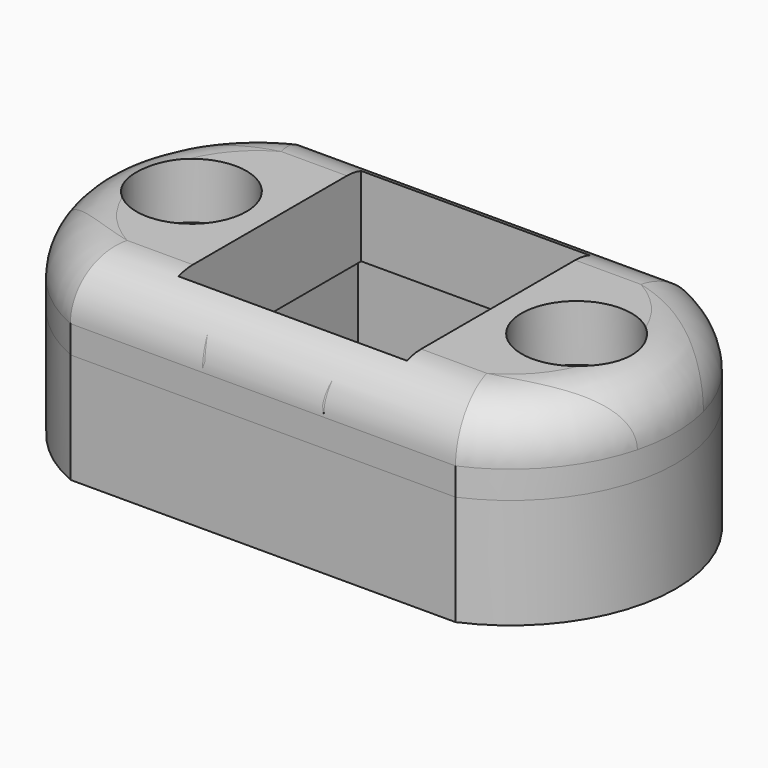
from build123d import *

# Parameters (mm, degrees)
F0_W           = 14
F0_H           = 11
F1_DEPTH       = 4
F2_R           = 1
F2_W           = 9.5
F2_H           = 9.5
F3_DEPTH       = 5
F4_W           = 14
F4_H           = 11
F5_DEPTH       = 3
F6_W           = 8.3
F6_H           = 8.3
F7_DEPTH       = 3
F8_T1_DEPTH    = 24
F8_T6_ANGLE    = 228.4636950683
F8_S7_R        = 2
F8_T8_DEPTH    = 9
F8_S9_R        = 2
F8_T10_DEPTH   = 9
F8_T14_ANGLE   = 228.4636950683
F8_T19_ANGLE   = 228.4636950683
F8_S20_R       = 2
F8_T21_DEPTH   = 9
F8_S22_R       = 2
F8_T23_DEPTH   = 9
F8_T27_ANGLE   = 228.4636950683
F9_D           = 2
F9_DEPTH       = 20
F9_START       = 0.039984
F9_CBORE_D     = 4
F9_CBORE_DEPTH = 2
F9_TIP         = 0.600860619


# Not quite as in the source:
# - a fillet or chamfer that OpenCascade refuses, or shapes differently, is made with other operations: its cross-section is extruded or revolved along the edge and cut away or added


with BuildPart() as f1:
    # F0 (on Top) → F1 (new body)
    with BuildSketch(Plane.XY):
        Rectangle(F0_W, F0_H)
        with BuildLine():
            ThreePointArc((7, -5.5), (10.6020842383, 0), (7, 5.5))
            Line((7, 5.5), (7, -5.5))
        make_face()
        with BuildLine():
            Line((-7, -5.5), (-7, 5.5))
            ThreePointArc((-7, 5.5), (-10.6020842383, 0), (-7, -5.5))
        make_face()
    extrude(amount=F1_DEPTH)

    # F2 (on face) → F3 (cut)
    with BuildSketch(Plane.XY.offset(4)):
        with Locations((-7, 0)):
            Circle(F2_R)
        with Locations((7, 0)):
            Circle(F2_R)
        Rectangle(F2_W, F2_H)
    extrude(amount=-F3_DEPTH, mode=Mode.SUBTRACT)


with BuildPart() as f5:
    # F4 (on face) → F5 (new body)
    with BuildSketch(Plane.XY.offset(4)):
        Rectangle(F4_W, F4_H)
        with BuildLine():
            ThreePointArc((7, -5.5), (10.6020842383, 0), (7, 5.5))
            Line((7, 5.5), (7, -5.5))
        make_face()
        with BuildLine():
            Line((-7, -5.5), (-7, 5.5))
            ThreePointArc((-7, 5.5), (-10.6020842383, 0), (-7, -5.5))
        make_face()
    extrude(amount=F5_DEPTH)

    # F6 (on face) → F7 (cut)
    with BuildSketch(Plane.XY.offset(7)):
        Rectangle(F6_W, F6_H)
    extrude(amount=-F7_DEPTH, mode=Mode.SUBTRACT)

    # F8: fillet of radius 2 on 4 edges, made by hand

    # F8_s2 → F8_t1 (cut)
    with BuildSketch(Plane.YZ.offset(-12)):
        with BuildLine():
            ThreePointArc((5.5, 5), (4.9142135624, 6.4142135624), (3.5, 7))
            Line((3.5, 7), (5.5, 7))
            Line((5.5, 7), (5.5, 5))
        make_face()
        with BuildLine():
            ThreePointArc((-3.5, 7), (-4.9142135624, 6.4142135624), (-5.5, 5))
            Line((-5.5, 5), (-5.5, 7))
            Line((-5.5, 7), (-3.5, 7))
        make_face()
    extrude(amount=F8_T1_DEPTH, mode=Mode.SUBTRACT)


with BuildPart() as f8_tool4:
    # F8_s5 → F8_t6 (revolve)
    with BuildSketch(Plane(origin=(3.8268504556, -1.7224121907, 0), x_dir=(0, 0, 1), z_dir=(-0.9118921219, 0.4104299673, 0))):
        with BuildLine():
            ThreePointArc((5, -4.1111667166), (6.4142135624, -3.525380279), (7, -2.1111667166))
            Line((7, -2.1111667166), (7, -4.1111667166))
            Line((7, -4.1111667166), (5, -4.1111667166))
        make_face()
    revolve(axis=Axis((4.6020842383, 0, 7), (0, 0, 1)), revolution_arc=F8_T6_ANGLE)

    # F8_s7 → F8_t8 (cut, symmetric)
    with BuildSketch(Plane.YZ.offset(6.3)):
        with Locations((3.5, 5)):
            Circle(F8_S7_R)
    extrude(amount=F8_T8_DEPTH, both=True, mode=Mode.SUBTRACT)

    # F8_s9 → F8_t10 (cut, symmetric)
    with BuildSketch(Plane.YZ.offset(6.3)):
        with Locations((-3.5, 5)):
            Circle(F8_S9_R)
    extrude(amount=F8_T10_DEPTH, both=True, mode=Mode.SUBTRACT)


with BuildPart() as f5_1:
    add(f5.part)

    # F8_t3: cut F8_tool4
    add(f8_tool4.part, mode=Mode.SUBTRACT)


with BuildPart() as f8_tool12:
    # F8_s13 → F8_t14 (revolve)
    with BuildSketch(Plane(origin=(3.8268504556, -1.7224121907, 0), x_dir=(0, 0, 1), z_dir=(-0.9118921219, 0.4104299673, 0))):
        with BuildLine():
            ThreePointArc((5, -4.1111667166), (6.4142135624, -3.525380279), (7, -2.1111667166))
            Line((7, -2.1111667166), (7, -4.1111667166))
            Line((7, -4.1111667166), (5, -4.1111667166))
        make_face()
    revolve(axis=Axis((4.6020842383, 0, 7), (0, 0, 1)), revolution_arc=F8_T14_ANGLE)

    split(bisect_by=Plane.YZ.offset(4.15), keep=Keep.TOP)


with BuildPart() as f5_2:
    add(f5_1.part)

    # F8_t11: cut F8_tool12
    add(f8_tool12.part, mode=Mode.SUBTRACT)


with BuildPart() as f8_tool17:
    # F8_s18 → F8_t19 (revolve)
    with BuildSketch(Plane(origin=(-3.8268504556, 1.7224121907, 0), x_dir=(0, 0, 1), z_dir=(0.9118921219, -0.4104299673, 0))):
        with BuildLine():
            ThreePointArc((5, -4.1111667166), (6.4142135624, -3.525380279), (7, -2.1111667166))
            Line((7, -2.1111667166), (7, -4.1111667166))
            Line((7, -4.1111667166), (5, -4.1111667166))
        make_face()
    revolve(axis=Axis((-4.6020842383, 0, 7), (0, 0, 1)), revolution_arc=F8_T19_ANGLE)

    # F8_s20 → F8_t21 (cut, symmetric)
    with BuildSketch(Plane.YZ.offset(-6.3)):
        with Locations((3.5, 5)):
            Circle(F8_S20_R)
    extrude(amount=F8_T21_DEPTH, both=True, mode=Mode.SUBTRACT)

    # F8_s22 → F8_t23 (cut, symmetric)
    with BuildSketch(Plane.YZ.offset(-6.3)):
        with Locations((-3.5, 5)):
            Circle(F8_S22_R)
    extrude(amount=F8_T23_DEPTH, both=True, mode=Mode.SUBTRACT)


with BuildPart() as f5_3:
    add(f5_2.part)

    # F8_t16: cut F8_tool17
    add(f8_tool17.part, mode=Mode.SUBTRACT)


with BuildPart() as f8_tool25:
    # F8_s26 → F8_t27 (revolve)
    with BuildSketch(Plane(origin=(-3.8268504556, 1.7224121907, 0), x_dir=(0, 0, 1), z_dir=(0.9118921219, -0.4104299673, 0))):
        with BuildLine():
            ThreePointArc((5, -4.1111667166), (6.4142135624, -3.525380279), (7, -2.1111667166))
            Line((7, -2.1111667166), (7, -4.1111667166))
            Line((7, -4.1111667166), (5, -4.1111667166))
        make_face()
    revolve(axis=Axis((-4.6020842383, 0, 7), (0, 0, 1)), revolution_arc=F8_T27_ANGLE)

    split(bisect_by=Plane.YZ.offset(-4.15), keep=Keep.BOTTOM)


with BuildPart() as f5_4:
    add(f5_3.part)

    # F8_t24: cut F8_tool25
    add(f8_tool25.part, mode=Mode.SUBTRACT)

    # F9
    # its depths count from where the whole tool has entered the part; down to there all is cleared
    with Locations(Plane.XY.offset(7).offset(-F9_START)):
        with Locations((7, 0), (-7, 0)):
            CounterBoreHole(F9_D / 2, F9_CBORE_D / 2, F9_CBORE_DEPTH, depth=F9_DEPTH)
            with Locations((0, 0, -(F9_DEPTH + F9_TIP / 2))):  # 118° drill point
                Cone(0, F9_D / 2, F9_TIP, mode=Mode.SUBTRACT)


solid = Compound([f1.part, f5_4.part])
